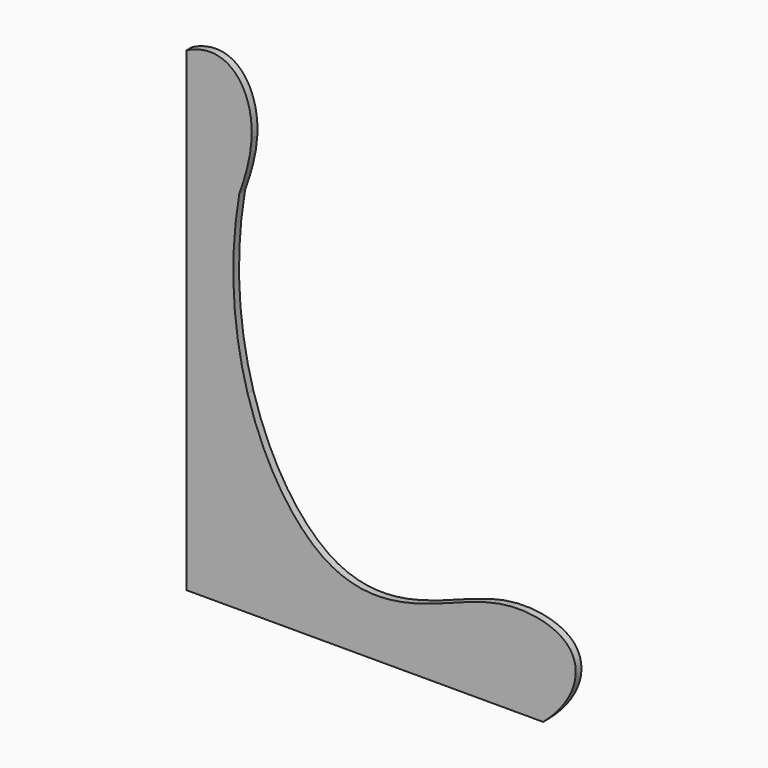
from build123d import *

# Parameters (mm, degrees)
F1_DEPTH = 3


with BuildPart() as f1:
    # F0 (on Front) → F1 (new body)
    with BuildSketch(Plane.XZ):
        with BuildLine():
            add(Edge.make_bspline(
                [(0, 200), (17.5350010591, 208.7052251042), (28.2990167117, 194.2533942124), (27.3598209023, 176.1217862368)],
                knots=[0, 0, 0, 0, 0.2121816796, 0.2121816796, 0.2121816796, 0.2121816796], degree=3))
            Line((0, 200), (0, 0))
            Line((0, 0), (150, 0))
            add(Edge.make_bspline(
                [(25.6660213946, 81.2246880313), (32.8761299375, 56.5068863186), (60.0117036649, 17.4585313325), (104.0532180707, 27.1280796833), (133.9334309453, 41.9003481082), (169.1529761494, 33.9703926018), (163.3473671479, 11.5198906648), (150, 0)],
                knots=[0.1766304626, 0.1766304626, 0.1766304626, 0.1766304626, 0.3437936291, 0.5310100844, 0.6957912123, 0.8398868931, 1, 1, 1, 1], degree=3))
            add(Edge.make_bspline(
                [(22.1886454738, 154.1668037154), (13.9805728557, 131.5466692926), (-6.7542086215, 97.2923947246), (17.0207337498, 84.6439779907), (25.666021385, 81.2246880244)],
                knots=[0.2931971005, 0.2931971005, 0.2931971005, 0.2931971005, 0.5352029466, 0.6440385187, 0.6440385187, 0.6440385187, 0.6440385187], degree=3))
            add(Edge.make_bspline(
                [(27.3598209023, 176.1217862368), (25.1275690328, 168.6815010828), (23.4215283398, 161.3493559456), (22.1886454738, 154.1668037154)],
                knots=[0, 0, 0, 0, 0.0368844878, 0.0368844878, 0.0368844878, 0.0368844878], degree=3))
        make_face()
        with BuildLine():
            add(Edge.make_bspline(
                [(27.3598209023, 176.1217862368), (27.0012162201, 169.1987575651), (24.9364322264, 161.7392642187), (22.1886454738, 154.1668037154)],
                knots=[0.2121816796, 0.2121816796, 0.2121816796, 0.2121816796, 0.2931971005, 0.2931971005, 0.2931971005, 0.2931971005], degree=3))
            add(Edge.make_bspline(
                [(27.3598209023, 176.1217862368), (25.1275690328, 168.6815010828), (23.4215283398, 161.3493559456), (22.1886454738, 154.1668037154)],
                knots=[0, 0, 0, 0, 0.0368844878, 0.0368844878, 0.0368844878, 0.0368844878], degree=3))
        make_face()
        with BuildLine():
            add(Edge.make_bspline(
                [(22.1886454738, 154.1668037154), (17.5175648086, 126.9539339651), (19.6384755701, 101.8884105841), (25.6660213946, 81.2246880313)],
                knots=[0.0368844878, 0.0368844878, 0.0368844878, 0.0368844878, 0.1766304626, 0.1766304626, 0.1766304626, 0.1766304626], degree=3))
            add(Edge.make_bspline(
                [(22.1886454738, 154.1668037154), (13.9805728557, 131.5466692926), (-6.7542086215, 97.2923947246), (17.0207337498, 84.6439779907), (25.666021385, 81.2246880244)],
                knots=[0.2931971005, 0.2931971005, 0.2931971005, 0.2931971005, 0.5352029466, 0.6440385187, 0.6440385187, 0.6440385187, 0.6440385187], degree=3))
        make_face()
    extrude(amount=F1_DEPTH)


solid = f1.part
